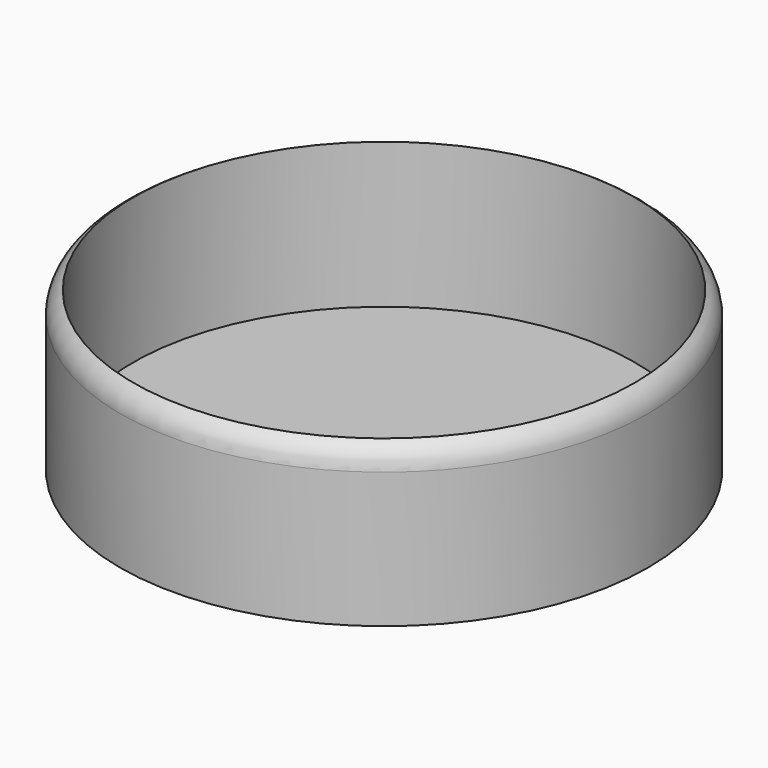
from build123d import *

# Parameters (mm, degrees)
F0_R     = 50
F1_DEPTH = 30
F2_T     = -2.5


# Not quite as in the source:
# - a fillet or chamfer that OpenCascade refuses, or shapes differently, is made with other operations: its cross-section is extruded or revolved along the edge and cut away or added


with BuildPart() as f1:
    # F0 (on Top) → F1 (new body)
    with BuildSketch(Plane.XY):
        Circle(F0_R)
    extrude(amount=F1_DEPTH)

    # F2
    f2_openings = [f1.faces().sort_by_distance(p)[0] for p in [
        (0, 0, 30),
    ]]
    offset(amount=F2_T, openings=f2_openings)

    # F3: fillet of radius 5 on 1 edges, made by hand

    # F3_s1 → F3_t2 (revolve, cut)
    with BuildSketch(Plane.XZ):
        with BuildLine():
            ThreePointArc((50, 25.6698729811), (49.3301270189, 28.1698729811), (47.5, 30))
            Line((47.5, 30), (50, 30))
            Line((50, 30), (50, 25.6698729811))
        make_face()
    revolve(axis=Axis((0, 0, 30), (0, 0, 1)), mode=Mode.SUBTRACT)


solid = f1.part
